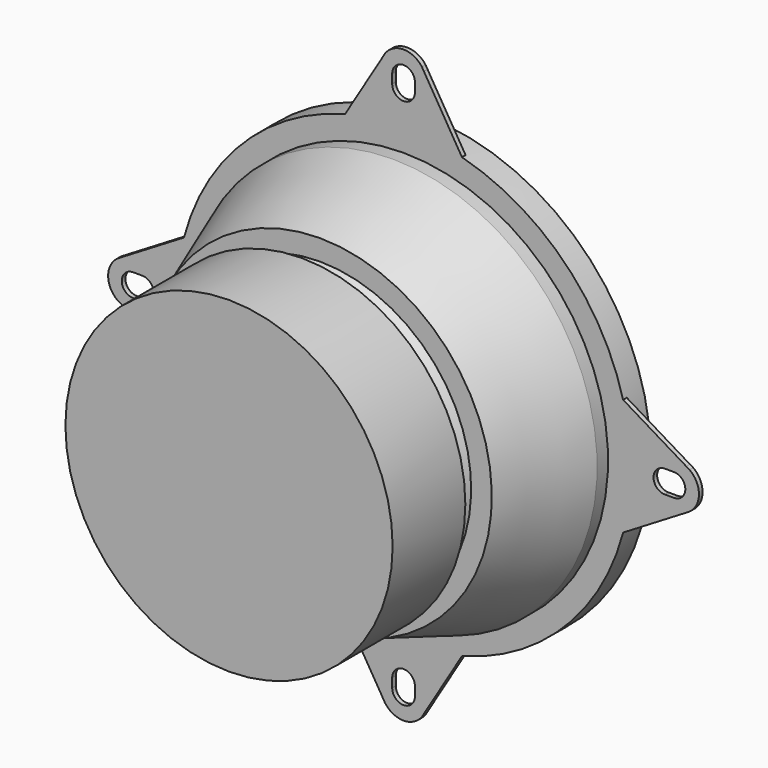
from build123d import *

# Parameters (mm, degrees)
F3_DEPTH = 1


with BuildPart() as f1:
    # F0 (on Right) → F1 (revolve)
    with BuildSketch(Plane.YZ):
        with BuildLine():
            Line((-61.0699225962, 0), (-22.4797911942, 0))
            Line((-22.4797911942, 0), (-11.0699225962, 38))
            ThreePointArc((-11.0699225962, 38), (-7.5699225962, 41.5), (-11.0699225962, 45))
            Line((-11.0699225962, 45), (-8.0699225962, 45))
            Line((-8.0699225962, 45), (-8.0699225962, 49))
            Line((-8.0699225962, 49), (-7.5699225962, 49))
            Line((-7.5699225962, 49), (-7.5699225962, 50))
            Line((-7.5699225962, 50), (-13.0699225962, 50))
            Line((-13.0699225962, 50), (-13.0699225962, 45))
            Line((-13.0699225962, 45), (-16.0699225962, 45))
            Line((-16.0699225962, 45), (-36.0699225962, 37.823528317))
            Line((-36.0699225962, 37.823528317), (-36.0699225962, 33.2837096231))
            Line((-36.0699225962, 33.2837096231), (-41.0699225962, 31.4013561058))
            Line((-41.0699225962, 31.4013561058), (-41.0699225962, 36))
            Line((-41.0699225962, 36), (-61.0699225962, 36))
            Line((-61.0699225962, 36), (-61.0699225962, 0))
        make_face()
    revolve(axis=Axis((0, -30.5349612981, 0), (0, -1, 0)))

    # F2 (on face) → F3 (join)
    with BuildSketch(Plane.XZ.offset(13.0699225962)):
        with BuildLine():
            Line((12.8560631669, 48.3189573547), (4.4851679108, 62.2098119404))
            Line((4.4851679108, 62.2098119404), (4.04924654, 62.9331898094))
            ThreePointArc((4.04924654, 62.9331898094), (0, 65), (-4.04924654, 62.9331898094))
            Line((-4.04924654, 62.9331898094), (-4.4851679108, 62.2098119404))
            Line((-4.4851679108, 62.2098119404), (-12.8560631669, 48.3189573547))
            ThreePointArc((-12.8560631669, 48.3189573547), (0, 50), (12.8560631669, 48.3189573547))
        make_face()
        with BuildLine():
            ThreePointArc((2.4997371633, 59.536250715), (2.5, 59.5), (2.4997371633, 59.463749285))
            Line((2.4997371633, 59.463749285), (2.4997371633, 57.536250715))
            ThreePointArc((2.4997371633, 57.536250715), (2.5, 57.5), (2.4997371633, 57.463749285))
            ThreePointArc((2.4997371633, 57.463749285), (0.0126154042, 55.0000318299), (-2.4992440087, 57.4385232966))
            ThreePointArc((-2.4992440087, 57.4385232966), (-2.5, 57.5), (-2.4992440087, 57.5614767034))
            Line((-2.4992440087, 57.5614767034), (-2.4992440087, 59.4385232966))
            ThreePointArc((-2.4992440087, 59.4385232966), (-2.5, 59.5), (-2.4992440087, 59.5614767034))
            ThreePointArc((-2.4992440087, 59.5614767034), (0.0126154042, 61.9999681701), (2.4997371633, 59.536250715))
        make_face(mode=Mode.SUBTRACT)
        with BuildLine():
            Line((62.2098119404, 4.4851679108), (48.3189573547, 12.8560631669))
            ThreePointArc((48.3189573547, 12.8560631669), (49.5779581454, 6.4827514322), (50, 0))
            ThreePointArc((50, 0), (49.5779581454, -6.4827514322), (48.3189573547, -12.8560631669))
            Line((48.3189573547, -12.8560631669), (62.2098119404, -4.4851679108))
            Line((62.2098119404, -4.4851679108), (62.9331898094, -4.04924654))
            ThreePointArc((62.9331898094, -4.04924654), (65, 0), (62.9331898094, 4.04924654))
            Line((62.9331898094, 4.04924654), (62.2098119404, 4.4851679108))
        make_face()
        with BuildLine():
            ThreePointArc((57.4385232966, 2.4992440087), (57.5, 2.5), (57.5614767034, 2.4992440087))
            Line((57.5614767034, 2.4992440087), (59.4385232966, 2.4992440087))
            ThreePointArc((59.4385232966, 2.4992440087), (59.5, 2.5), (59.5614767034, 2.4992440087))
            ThreePointArc((59.5614767034, 2.4992440087), (61.9999681701, -0.0126154042), (59.536250715, -2.4997371633))
            ThreePointArc((59.536250715, -2.4997371633), (59.5, -2.5), (59.463749285, -2.4997371633))
            Line((59.463749285, -2.4997371633), (57.536250715, -2.4997371633))
            ThreePointArc((57.536250715, -2.4997371633), (57.5, -2.5), (57.463749285, -2.4997371633))
            ThreePointArc((57.463749285, -2.4997371633), (55.0000318299, -0.0126154042), (57.4385232966, 2.4992440087))
        make_face(mode=Mode.SUBTRACT)
        with BuildLine():
            ThreePointArc((-48.3189573547, -12.8560631669), (-50, 0), (-48.3189573547, 12.8560631669))
            Line((-48.3189573547, 12.8560631669), (-62.2098119404, 4.4851679108))
            Line((-62.2098119404, 4.4851679108), (-62.9331898094, 4.04924654))
            ThreePointArc((-62.9331898094, 4.04924654), (-65, 0), (-62.9331898094, -4.04924654))
            Line((-62.9331898094, -4.04924654), (-62.2098119404, -4.4851679108))
            Line((-62.2098119404, -4.4851679108), (-48.3189573547, -12.8560631669))
        make_face()
        with BuildLine():
            ThreePointArc((-57.4385232966, -2.4992440087), (-57.5, -2.5), (-57.5614767034, -2.4992440087))
            Line((-57.5614767034, -2.4992440087), (-59.4385232966, -2.4992440087))
            ThreePointArc((-59.4385232966, -2.4992440087), (-59.5, -2.5), (-59.5614767034, -2.4992440087))
            ThreePointArc((-59.5614767034, -2.4992440087), (-61.9999681701, 0.0126154042), (-59.536250715, 2.4997371633))
            ThreePointArc((-59.536250715, 2.4997371633), (-59.5, 2.5), (-59.463749285, 2.4997371633))
            Line((-59.463749285, 2.4997371633), (-57.536250715, 2.4997371633))
            ThreePointArc((-57.536250715, 2.4997371633), (-57.5, 2.5), (-57.463749285, 2.4997371633))
            ThreePointArc((-57.463749285, 2.4997371633), (-55.0000318299, 0.0126154042), (-57.4385232966, -2.4992440087))
        make_face(mode=Mode.SUBTRACT)
        with BuildLine():
            Line((4.4851679108, -62.2098119404), (12.8560631669, -48.3189573547))
            ThreePointArc((12.8560631669, -48.3189573547), (0, -50), (-12.8560631669, -48.3189573547))
            Line((-12.8560631669, -48.3189573547), (-4.4851679108, -62.2098119404))
            Line((-4.4851679108, -62.2098119404), (-4.04924654, -62.9331898094))
            ThreePointArc((-4.04924654, -62.9331898094), (0, -65), (4.04924654, -62.9331898094))
            Line((4.04924654, -62.9331898094), (4.4851679108, -62.2098119404))
        make_face()
        with BuildLine():
            ThreePointArc((2.4992440087, -57.4385232966), (2.5, -57.5), (2.4992440087, -57.5614767034))
            Line((2.4992440087, -57.5614767034), (2.4992440087, -59.4385232966))
            ThreePointArc((2.4992440087, -59.4385232966), (2.5, -59.5), (2.4992440087, -59.5614767034))
            ThreePointArc((2.4992440087, -59.5614767034), (-0.0126154042, -61.9999681701), (-2.4997371633, -59.536250715))
            ThreePointArc((-2.4997371633, -59.536250715), (-2.5, -59.5), (-2.4997371633, -59.463749285))
            Line((-2.4997371633, -59.463749285), (-2.4997371633, -57.536250715))
            ThreePointArc((-2.4997371633, -57.536250715), (-2.5, -57.5), (-2.4997371633, -57.463749285))
            ThreePointArc((-2.4997371633, -57.463749285), (-0.0126154042, -55.0000318299), (2.4992440087, -57.4385232966))
        make_face(mode=Mode.SUBTRACT)
    extrude(amount=-F3_DEPTH)


solid = f1.part
